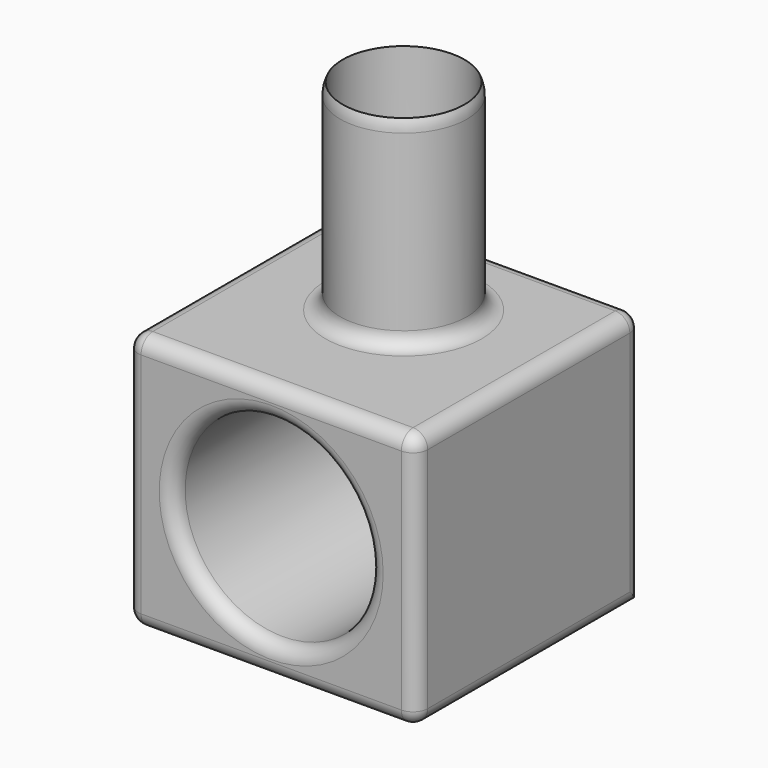
from build123d import *

# Parameters (mm, degrees)
F0_W     = 100.4092097282
F0_H     = 89.206546545
F1_DEPTH = 97.7773964405
F2_R     = 22.0167060196
F2_R_2   = 21.115809679
F3_DEPTH = 114.1652464867
F4_R     = 5.08
F5_R     = 33.8357748328
F6_DEPTH = 98.3386710286
F7_R     = 5


# Not quite as in the source:
# - a fillet or chamfer that OpenCascade refuses, or shapes differently, is made with other operations: its cross-section is extruded or revolved along the edge and cut away or added
# - the program builds the solid bodies; features that only make, move or delete a surface that nothing else refers to are left out


with BuildPart() as f1:
    # F0 (on Front) → F1 (new body)
    with BuildSketch(Plane.XZ):
        Rectangle(F0_W, F0_H)
    extrude(amount=F1_DEPTH)

    # F2 (on Top) → F3 (join)
    with BuildSketch(Plane.XY):
        with Locations((0, -40.3943955898)):
            Circle(F2_R)
        with Locations((0, -40.3943955898)):
            Circle(F2_R_2, mode=Mode.SUBTRACT)
    extrude(amount=F3_DEPTH)

    # F4
    f4_edges = [f1.edges().sort_by_distance(p)[0] for p in [
        (50.204605, -48.888698, 44.603273),
        (0, 0, 44.603273),
        (0, -97.777396, 44.603273),
        (-50.204605, -48.888698, 44.603273),
        (-22.016706, -40.394396, 44.603273),
        (0, -97.777396, -44.603273),
        (50.204605, -97.777396, 0),
        (-50.204605, -97.777396, 0),
        (-50.204605, -48.888698, -44.603273),
        (-50.204605, 0, 0),
        (50.204605, -48.888698, -44.603273),
        (50.204605, 0, 0),
    ]]
    fillet(f4_edges, radius=F4_R)

    # F5 (on Front) → F6 (cut)
    with BuildSketch(Plane.XZ):
        Circle(F5_R)
    extrude(amount=F6_DEPTH, mode=Mode.SUBTRACT)

    # F7
    f7_edges = [f1.edges().sort_by_distance(p)[0] for p in [
        (50.204605, -48.888698, 39.523273),
        (50.204605, -5.08, 0),
        (50.204605, -92.697396, 0),
        (50.204605, -48.888698, -39.523273),
        (-33.835775, -97.777396, 0),
    ]]
    fillet(f7_edges, radius=F7_R)

    # F10: fillet of radius 10 on 1 edges, made by hand

    # F10_s1 → F10_t2 (revolve, cut)
    with BuildSketch(Plane.XZ.offset(40.3943955898)):
        with BuildLine():
            ThreePointArc((22.0167060196, 110.017197235), (21.7888868559, 112.1395736631), (21.115809679, 114.1652464867))
            Line((21.115809679, 114.1652464867), (22.0167060196, 114.1652464867))
            Line((22.0167060196, 114.1652464867), (22.0167060196, 110.017197235))
        make_face()
    revolve(axis=Axis((0, -40.3943955898, 114.1652464867), (0, 0, 1)), mode=Mode.SUBTRACT)


solid = f1.part
